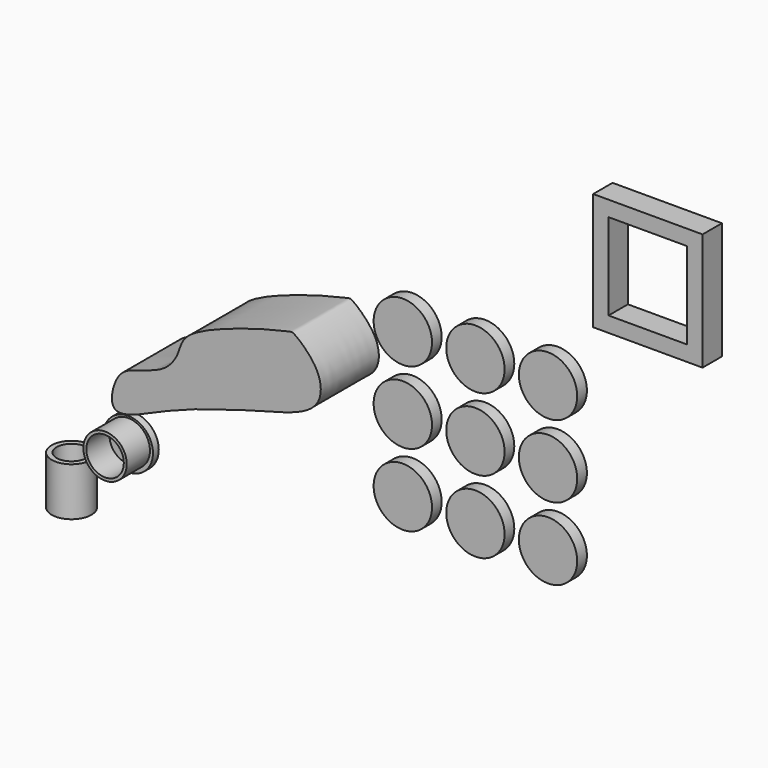
from build123d import *

# Parameters (mm, degrees)
F0_R      = 82.1326203769
F0_R_2    = 61.4272879331
F1_DEPTH  = 200
F2_R      = 71.5377696559
F3_DEPTH  = 30
F4_R      = 89.524835576
F4_R_2    = 77.5158713494
F5_DEPTH  = 150
F6_R      = 102.6083377999
F7_DEPTH  = 30
F9_DEPTH  = 300
F10_R     = 120.562503411
F11_DEPTH = 50
F12_W     = 451.8953561783
F12_H     = 484.7009181976
F12_W_2   = 324.9243497849
F12_H_2   = 357.7299118042
F13_DEPTH = 100


with BuildPart() as f1:
    # F0 (on Top) → F1 (new body)
    with BuildSketch(Plane.XY):
        with Locations((-287.736415863, -110.3699430823)):
            Circle(F0_R)
        with Locations((-287.736415863, -110.3699430823)):
            Circle(F0_R_2, mode=Mode.SUBTRACT)
    extrude(amount=F1_DEPTH)

    # F2 (on Top) → F3 (join)
    with BuildSketch(Plane.XY):
        with Locations((-288.881868124, -110.3232502937)):
            Circle(F2_R)
    extrude(amount=F3_DEPTH)


with BuildPart() as f5:
    # F4 (on Front) → F5 (new body)
    with BuildSketch(Plane.XZ):
        with Locations((-117.5889223814, 258.5912942886)):
            Circle(F4_R)
        with Locations((-117.5889223814, 258.5912942886)):
            Circle(F4_R_2, mode=Mode.SUBTRACT)
    extrude(amount=F5_DEPTH)

    # F6 (on Front) → F7 (join)
    with BuildSketch(Plane.XZ):
        with Locations((-118.300832808, 253.4432709217)):
            Circle(F6_R)
    extrude(amount=F7_DEPTH)


with BuildPart() as f9:
    # F8 (on Front) → F9 (new body)
    with BuildSketch(Plane.XZ):
        with BuildLine():
            add(Edge.make_bspline(
                [(57.3537684977, 665.344953537), (75.7396222507, 693.1721150366), (120.441491181, 709.5448357572), (181.4797555431, 728.1579200138), (256.7638546749, 754.7876508309), (313.3576484638, 831.5283338475), (319.4403702514, 945.7132685504), (763.8351652874, 1063.7268843019), (783.8687718693, 1059.89713934), (897.0662056264, 966.5278160698), (904.7858656689, 795.6260859729), (654.2885118019, 736.6125697023), (485.8516571578, 685.1996083758), (270.9847120753, 620.5528684155), (-0.632949876, 478.4268568096), (34.3286446619, 630.4962134058), (57.3537684977, 665.344953537)],
                knots=[0, 0, 0, 0, 0.0537973226, 0.1021445662, 0.1559707325, 0.2122728407, 0.2745998963, 0.4004197393, 0.4313636464, 0.5009271471, 0.5716108321, 0.6632436084, 0.7460616771, 0.842301151, 0.9326280938, 1, 1, 1, 1], degree=3))
        make_face()
    extrude(amount=F9_DEPTH)


with BuildPart() as f11:
    # F10 (on Front) → F11 (new body)
    with BuildSketch(Plane.XZ):
        with Locations((1032.5639247894, 444.2869126797)):
            Circle(F10_R)
    extrude(amount=F11_DEPTH)


with BuildPart() as f11b:
    # F10 (on Front) → F11, piece 2 (new body)
    with BuildSketch(Plane.XZ):
        with Locations((1032.5639247894, 744.2869126797)):
            Circle(F10_R)
    extrude(amount=F11_DEPTH)


with BuildPart() as f11c:
    # F10 (on Front) → F11, piece 3 (new body)
    with BuildSketch(Plane.XZ):
        with Locations((1032.5639247894, 1044.2869126797)):
            Circle(F10_R)
    extrude(amount=F11_DEPTH)


with BuildPart() as f11d:
    # F10 (on Front) → F11, piece 4 (new body)
    with BuildSketch(Plane.XZ):
        with Locations((1332.5639247894, 444.2869126797)):
            Circle(F10_R)
    extrude(amount=F11_DEPTH)


with BuildPart() as f11e:
    # F10 (on Front) → F11, piece 5 (new body)
    with BuildSketch(Plane.XZ):
        with Locations((1332.5639247894, 744.2869126797)):
            Circle(F10_R)
    extrude(amount=F11_DEPTH)


with BuildPart() as f11f:
    # F10 (on Front) → F11, piece 6 (new body)
    with BuildSketch(Plane.XZ):
        with Locations((1332.5639247894, 1044.2869126797)):
            Circle(F10_R)
    extrude(amount=F11_DEPTH)


with BuildPart() as f11g:
    # F10 (on Front) → F11, piece 7 (new body)
    with BuildSketch(Plane.XZ):
        with Locations((1632.5639247894, 444.2869126797)):
            Circle(F10_R)
    extrude(amount=F11_DEPTH)


with BuildPart() as f11h:
    # F10 (on Front) → F11, piece 8 (new body)
    with BuildSketch(Plane.XZ):
        with Locations((1632.5639247894, 744.2869126797)):
            Circle(F10_R)
    extrude(amount=F11_DEPTH)


with BuildPart() as f11i:
    # F10 (on Front) → F11, piece 9 (new body)
    with BuildSketch(Plane.XZ):
        with Locations((1632.5639247894, 1044.2869126797)):
            Circle(F10_R)
    extrude(amount=F11_DEPTH)


with BuildPart() as f13:
    # F12 (on Front) → F13 (new body)
    with BuildSketch(Plane.XZ):
        with Locations((2084.9931836128, 1591.9594764709)):
            Rectangle(F12_W, F12_H)
        with Locations((2084.9931836128, 1591.9594764709)):
            Rectangle(F12_W_2, F12_H_2, mode=Mode.SUBTRACT)
    extrude(amount=F13_DEPTH)


solid = Compound([f1.part, f5.part, f9.part, f11.part, f11b.part, f11c.part, f11d.part, f11e.part, f11f.part, f11g.part, f11h.part, f11i.part, f13.part])
